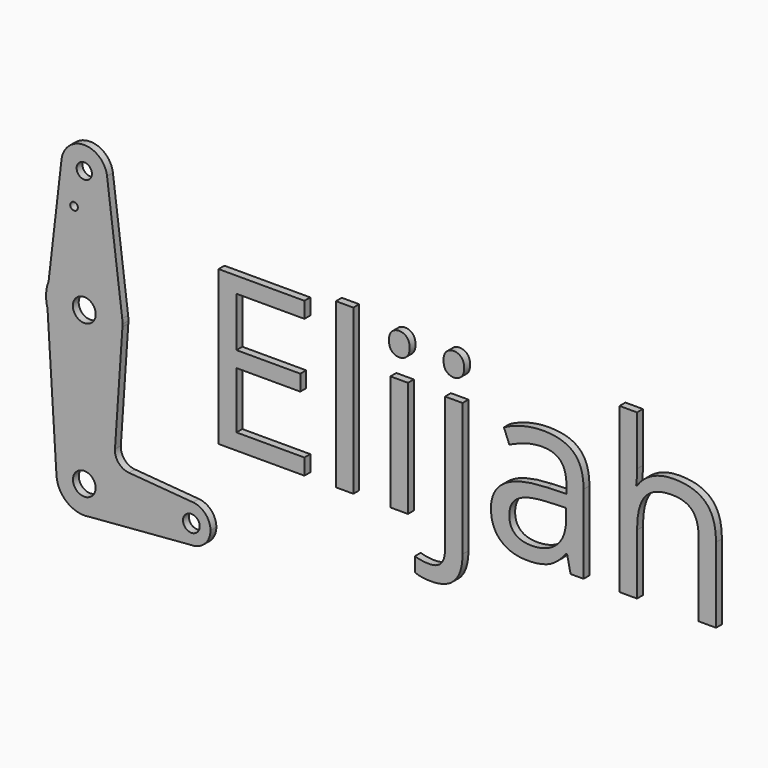
from build123d import *

# Parameters (mm, degrees)
F0_R         = 3.175
F0_R_2       = 1.5875
F0_R_3       = 4.7575068097
F0_R_4       = 4.7051210797
F0_R_5       = 3.4618536907
F0_TEXT_SIZE = 89.5419002821
F1_DEPTH     = 3.048


# Not quite as in the source:
# - Text() gives the source's letters only with a copy of the font that has no kerning and outlines rounded to 1/6400 em; it was checked with that copy


with BuildPart() as f1:
    # F0 (on Front) → F1 (new body)
    with BuildSketch(Plane.XZ):
        with BuildLine():
            ThreePointArc((-62.3327647056, 62.6235962344), (-53.419168339, 52.0196425515), (-43.3458857198, 61.5288492045))
            ThreePointArc((-43.3458857198, 61.5288492045), (-43.3645808256, 62.1253324464), (-43.4205927556, 62.7194742045))
            ThreePointArc((-43.4205927556, 62.7194742045), (-52.9191734539, 71.0537268044), (-62.3327647056, 62.6235962344))
        make_face()
        with Locations((-52.8708857198, 61.5288492045)):
            Circle(F0_R, mode=Mode.SUBTRACT)
        with BuildLine():
            ThreePointArc((-43.4205927556, 62.7194742045), (-43.3645808256, 62.1253324464), (-43.3458857198, 61.5288492045))
            ThreePointArc((-43.3458857198, 61.5288492045), (-53.419168339, 52.0196425515), (-62.3327647056, 62.6235962344))
            Line((-62.3327647056, 62.6235962344), (-67.6733629439, 16.4649012467))
            ThreePointArc((-67.6733629439, 16.4649012467), (-50.9360856281, 26.4855041034), (-37.1203974462, 12.7132242045))
            Line((-37.1203974462, 12.7132242045), (-43.4205927556, 62.7194742045))
        make_face()
        with Locations((-57.121746242, 47.2540492045)):
            Circle(F0_R_2, mode=Mode.SUBTRACT)
        with BuildLine():
            ThreePointArc((-36.9958857198, 10.7288492045), (-37.0270442295, 11.7229879411), (-37.1203974462, 12.7132242045))
            ThreePointArc((-37.1203974462, 12.7132242045), (-50.9360856281, 26.4855041034), (-67.6733629439, 16.4649012467))
            ThreePointArc((-67.6733629439, 16.4649012467), (-68.7286214731, 11.4690125511), (-68.143305495, 6.3965496751))
            ThreePointArc((-68.143305495, 6.3965496751), (-51.2191636833, -5.0599898698), (-37.03250849, 9.6511517865))
            ThreePointArc((-37.03250849, 9.6511517865), (-37.0050440541, 10.1896894526), (-36.9958857198, 10.7288492045))
        make_face()
        with Locations((-52.8708857198, 10.7288492045)):
            Circle(F0_R_3, mode=Mode.SUBTRACT)
        with BuildLine():
            ThreePointArc((-37.03250849, 9.6511517865), (-51.2191636833, -5.0599898698), (-68.143305495, 6.3965496751))
            Line((-68.143305495, 6.3965496751), (-64.4127234272, -53.4901381753))
            ThreePointArc((-64.4127234272, -53.4901381753), (-53.230553409, -41.2125349758), (-41.3066753917, -52.7711507955))
            ThreePointArc((-41.3066753917, -52.7711507955), (-44.055867972, -60.2562307964), (-50.9962989853, -64.1824121233))
            Line((-50.9962989853, -64.1824121233), (-8.4208857198, -60.7086507955))
            ThreePointArc((-8.4208857198, -60.7086507955), (-16.3519042584, -52.4504465843), (-7.7800010471, -44.8595660563))
            Line((-7.7800010471, -44.8595660563), (-34.3127179869, -42.7102606802))
            ThreePointArc((-34.3127179869, -42.7102606802), (-38.6114080523, -40.5250188511), (-40.1353611406, -35.9499139217))
            Line((-40.1353611406, -35.9499139217), (-37.03250849, 9.6511517865))
        make_face()
        with BuildLine():
            ThreePointArc((-41.3066753917, -52.7711507955), (-53.230553409, -41.2125349758), (-64.4127234272, -53.4901381753))
            ThreePointArc((-64.4127234272, -53.4901381753), (-60.7897378851, -61.1986498848), (-52.8708857198, -64.3353611237))
            Line((-52.8708857198, -64.3353611237), (-50.9962989853, -64.1824121233))
            ThreePointArc((-50.9962989853, -64.1824121233), (-44.055867972, -60.2562307964), (-41.3066753917, -52.7711507955))
        make_face()
        with Locations((-52.8708857198, -52.7711507955)):
            Circle(F0_R_4, mode=Mode.SUBTRACT)
        with BuildLine():
            Line((-50.9962989853, -64.1824121233), (-52.8708857198, -64.3353611237))
            ThreePointArc((-52.8708857198, -64.3353611237), (-51.9304777204, -64.2970604477), (-50.9962989853, -64.1824121233))
        make_face()
        with BuildLine():
            ThreePointArc((-0.4833857198, -52.7711507955), (-2.586036607, -47.3898459278), (-7.7800010471, -44.8595660563))
            ThreePointArc((-7.7800010471, -44.8595660563), (-16.3519042584, -52.4504465843), (-8.4208857198, -60.7086507955))
            ThreePointArc((-8.4208857198, -60.7086507955), (-2.8082256442, -58.3838108712), (-0.4833857198, -52.7711507955))
        make_face()
        with Locations((-8.4208857198, -52.7711507955)):
            Circle(F0_R_5, mode=Mode.SUBTRACT)
        with Locations((-5.9225261211, -20.1033353806)):
            Text('Elijah', F0_TEXT_SIZE, font='Open Sans', text_align=(TextAlign.LEFT, TextAlign.BOTTOM))
    extrude(amount=F1_DEPTH)


solid = f1.part
